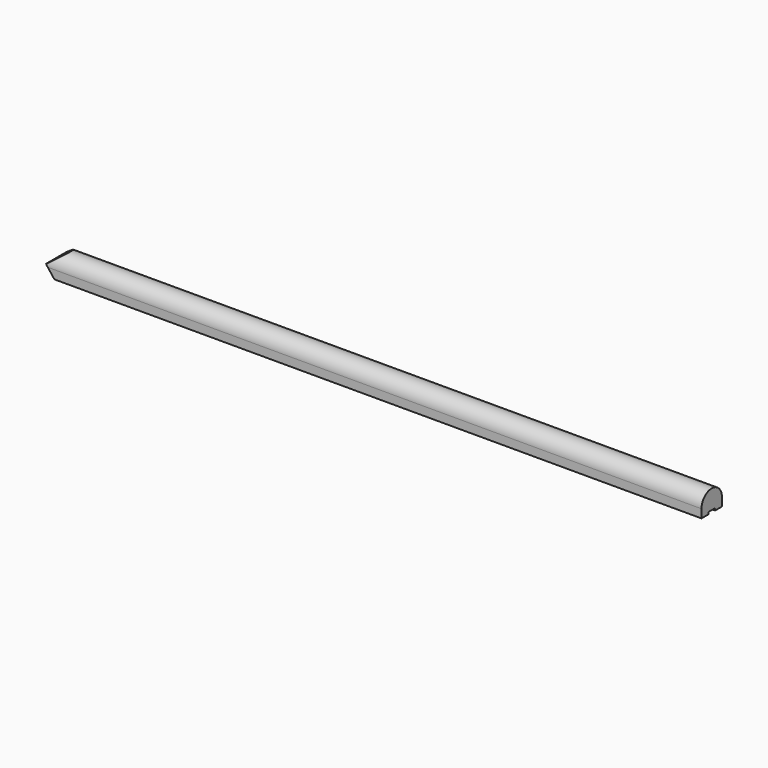
from build123d import *

# Parameters (mm, degrees)
F1_DEPTH = 1955.8
F2_SIZE2 = 32.5105174577
F2_SIZE  = 25.4
F4_DEPTH = 76.201


# Not quite as in the source:
# - a feature names something its author has since deleted; it is built from what else it names


with BuildPart() as f1:
    # F0 (on Right) → F1 (new body)
    with BuildSketch(Plane.YZ):
        with BuildLine():
            Line((0, 0), (0, -25.4))
            Line((0, -25.4), (25.4, -25.4))
            Line((25.4, -25.4), (25.4, -19.05))
            Line((25.4, -19.05), (50.8, -19.05))
            Line((50.8, -19.05), (50.8, -25.4))
            Line((50.8, -25.4), (76.2, -25.4))
            Line((76.2, -25.4), (76.2, 0))
            ThreePointArc((76.2, 0), (38.1, 38.1), (0, 0))
        make_face()
    extrude(amount=F1_DEPTH)

    # F2
    f2_edges = [f1.edges().sort_by_distance(p)[0] for p in [
        (0, 12.7, -25.4),
    ]]
    f2_side = f1.faces().sort_by_distance((977.9, 12.7, -25.4))[0]
    chamfer(f2_edges, length=F2_SIZE, length2=F2_SIZE2, reference=f2_side)

    # F3 (on Front) → F4 (cut, through all)
    with BuildSketch(Plane.XZ):
        Polygon((44.9116937816, 39.251241833), (17.98238638, 50.449128889), (0, 45.5416738987), (0, 7.1105174577), align=None)
    extrude(amount=-F4_DEPTH, mode=Mode.SUBTRACT)


solid = f1.part
